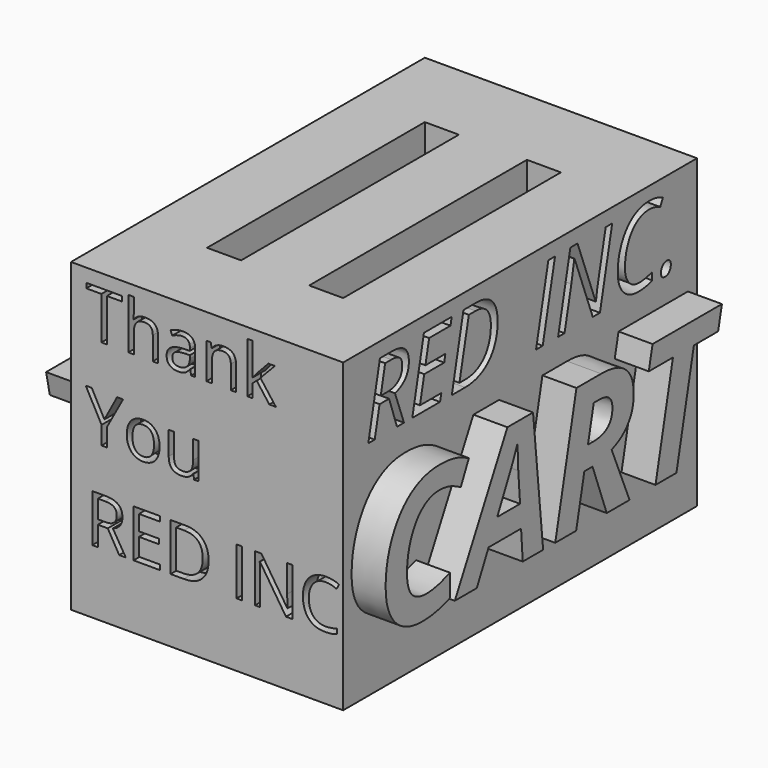
from build123d import *

# Parameters (mm, degrees)
F0_W            = 25.4
F0_H            = 25.4
F1_DEPTH        = 82.55
F2_W            = 25.4
F2_H            = 25.4
F3_DEPTH        = 165.1
F4_W            = 31.75
F4_H            = 25.4
F5_DEPTH        = 101.6
F6_TEXT_SIZE    = 65.6298136646
F7_DEPTH        = 12.7
F8_TEXT_SIZE    = 65.6298136646
F9_DEPTH        = 12.7
F10_TEXT_SIZE   = 39.687501784
F10_TEXT_SIZE_2 = 37.1619321716
F11_DEPTH       = 12.7
F12_TEXT_SIZE   = 36.0795503689
F12_TEXT_SIZE_2 = 37.883524783
F13_DEPTH       = 12.7
F14_W           = 101.6
F14_H           = 165.1
F15_DEPTH       = 25.4
F16_TEXT_SIZE   = 24.8948836492
F17_DEPTH       = 6.35
F18_TEXT_SIZE   = 20.2045465509
F19_DEPTH       = 6.35


# Not quite as in the source:
# - Text() gives the source's letters only with a copy of the font that has no kerning and outlines rounded to 1/6400 em; it was checked with that copy


with BuildPart() as f1:
    # F0 (on Front) → F1 (new body, symmetric)
    with BuildSketch(Plane.XZ):
        Polygon((-12.7, 45.2315360476), (-38.1, 45.2315360476), (-38.1, -43.6684639524), (0, -43.6684639524), (0, 19.8315360476), (-12.7, 19.8315360476), align=None)
        Polygon((0, 19.8315360476), (0, -43.6684639524), (63.5, -43.6684639524), (63.5, 19.8315360476), (38.1, 19.8315360476), align=None)
        with Locations((50.8, 32.5315360476)):
            Rectangle(F0_W, F0_H)
    extrude(amount=F1_DEPTH, both=True)

    # F2 (on face) → F3 (join)
    with BuildSketch(Plane.XZ.offset(82.55)):
        with Locations((12.7, 32.5315360476)):
            Rectangle(F2_W, F2_H)
    extrude(amount=-F3_DEPTH)

    # F4 (on face) → F5 (join)
    with BuildSketch(Plane.YZ.offset(63.5)):
        with Locations((-66.675, 32.5315360476)):
            Rectangle(F4_W, F4_H)
        with Locations((66.675, 32.5315360476)):
            Rectangle(F4_W, F4_H)
    extrude(amount=-F5_DEPTH)

    # F6 (on face) → F7 (join)
    with BuildSketch(Plane(origin=(-38.1, 0, 0), x_dir=(0, -1, 0), z_dir=(-1, 0, 0))):
        with Locations((-82.55, -43.6684639524)):
            Text('CART', F6_TEXT_SIZE, font='Open Sans', font_style=FontStyle.BOLDITALIC, text_align=(TextAlign.LEFT, TextAlign.BOTTOM))
    extrude(amount=F7_DEPTH)

    # F8 (on face) → F9 (join)
    with BuildSketch(Plane.YZ.offset(63.5)):
        with Locations((-82.55, -43.6684639524)):
            Text('CART', F8_TEXT_SIZE, font='Open Sans', font_style=FontStyle.BOLDITALIC, text_align=(TextAlign.LEFT, TextAlign.BOTTOM))
    extrude(amount=F9_DEPTH)

    # F10 (on face) → F11 (cut)
    with BuildSketch(Plane(origin=(-38.1, 0, 0), x_dir=(0, -1, 0), z_dir=(-1, 0, 0))):
        with Locations((-80.1398903131, 14.1576137394)):
            Text('RED', F10_TEXT_SIZE, font='Open Sans', font_style=FontStyle.ITALIC, text_align=(TextAlign.LEFT, TextAlign.BOTTOM))
        with Locations((4.0264772251, 14.9369323626)):
            Text('INC.', F10_TEXT_SIZE_2, font='Open Sans', text_align=(TextAlign.LEFT, TextAlign.BOTTOM))
    extrude(amount=-F11_DEPTH, mode=Mode.SUBTRACT)

    # F12 (on face) → F13 (cut)
    with BuildSketch(Plane.YZ.offset(63.5)):
        with Locations((-72.346707806, 13.8978417963)):
            Text('RED', F12_TEXT_SIZE, font='Open Sans', font_style=FontStyle.ITALIC, text_align=(TextAlign.LEFT, TextAlign.BOTTOM))
        with Locations((5.8448854834, 12.8587502986)):
            Text('INC.', F12_TEXT_SIZE_2, font='Open Sans', font_style=FontStyle.ITALIC, text_align=(TextAlign.LEFT, TextAlign.BOTTOM))
    extrude(amount=-F13_DEPTH, mode=Mode.SUBTRACT)

    # F14 (on face) → F15 (join)
    with BuildSketch(Plane(origin=(0, 0, -43.6684639524), x_dir=(1, 0, 0), z_dir=(0, 0, -1))):
        with Locations((12.7, 0)):
            Rectangle(F14_W, F14_H)
    extrude(amount=F15_DEPTH)

    # F16 (on face) → F17 (cut)
    with BuildSketch(Plane.XZ.offset(82.55)):
        with Locations((-32.6014794409, 22.4703401327)):
            Text('Thank', F16_TEXT_SIZE, font='Open Sans', text_align=(TextAlign.LEFT, TextAlign.BOTTOM))
        with Locations((-32.6014794409, -11.3867016302)):
            Text('You', F16_TEXT_SIZE, font='Open Sans', text_align=(TextAlign.LEFT, TextAlign.BOTTOM))
        with Locations((-32.6014794409, -45.2437433932)):
            Text('RED INC.', F16_TEXT_SIZE, font='Open Sans', text_align=(TextAlign.LEFT, TextAlign.BOTTOM))
    extrude(amount=-F17_DEPTH, mode=Mode.SUBTRACT)

    # F18 (on face) → F19 (cut)
    with BuildSketch(Plane(origin=(0, 82.55, 0), x_dir=(-1, 0, 0), z_dir=(0, 1, 0))):
        with Locations((-55.4614812136, 21.9507981092)):
            Text('Thank', F18_TEXT_SIZE, font='Open Sans', text_align=(TextAlign.LEFT, TextAlign.BOTTOM))
        with Locations((-55.4614812136, -5.5273852001)):
            Text('You', F18_TEXT_SIZE, font='Open Sans', text_align=(TextAlign.LEFT, TextAlign.BOTTOM))
        with Locations((-55.4614812136, -33.0055685093)):
            Text('RED INC', F18_TEXT_SIZE, font='Open Sans', text_align=(TextAlign.LEFT, TextAlign.BOTTOM))
    extrude(amount=-F19_DEPTH, mode=Mode.SUBTRACT)


solid = f1.part
